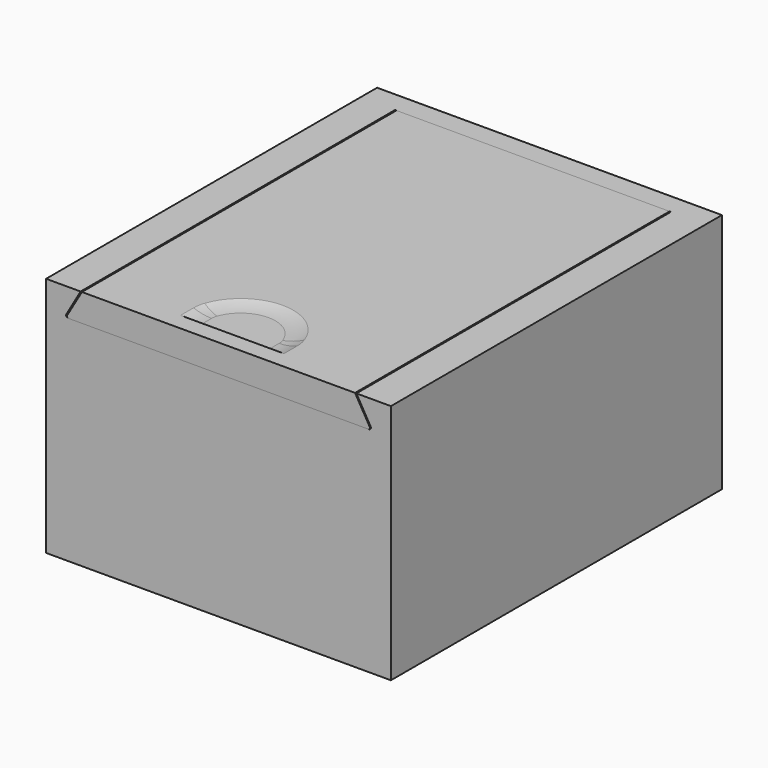
from build123d import *

# Parameters (mm, degrees)
F1_DEPTH      = 30
F1_DEPTH_BACK = 30
F2_W          = 40
F2_H          = 26
F3_DEPTH      = 3
F5_DEPTH      = 3
F6_DEPTH      = 30
F6_DEPTH_BACK = 27
F8_DEPTH      = 0.5
F9_T1_DEPTH   = 2.3744754405
F9_T4_ANGLE   = 141.4413290381
F9_T6_ANGLE   = 19.2793354809
F9_T8_ANGLE   = 19.2793354809


# Not quite as in the source:
# - a fillet or chamfer that OpenCascade refuses, or shapes differently, is made with other operations: its cross-section is extruded or revolved along the edge and cut away or added


with BuildPart() as f1:
    # F0 (on Front) → F1 (new body, two sides)
    with BuildSketch(Plane.XZ) as f1_sk:
        with BuildLine():
            Line((-25, -15), (0, -15))
            Line((0, -15), (0, -10))
            Line((0, -10), (-20, -10))
            Line((-20, -10), (-20, 15.9987840325))
            Line((-20, 15.9987840325), (-20, 16))
            Line((-20, 16), (-21.7897858345, 16))
            ThreePointArc((-21.7897858345, 16), (-22.0495934556, 16.15), (-22.0495934556, 16.45))
            Line((-22.0495934556, 16.45), (-20, 20))
            Line((-20, 20), (-25, 20))
            Line((-25, 20), (-25, -15))
        make_face()
        with BuildLine():
            Line((0, -10), (0, -15))
            Line((0, -15), (25, -15))
            Line((25, -15), (25, 20))
            Line((25, 20), (20, 20))
            Line((20, 20), (22.0495934556, 16.45))
            ThreePointArc((22.0495934556, 16.45), (22.0495934556, 16.15), (21.7897858345, 16))
            Line((21.7897858345, 16), (20, 16))
            Line((20, 16), (20, 15.9987840325))
            Line((20, 15.9987840325), (20, -10))
            Line((20, -10), (0, -10))
        make_face()
    extrude(amount=-F1_DEPTH)
    extrude(f1_sk.sketch, amount=F1_DEPTH_BACK)

    # F2 (on face) → F3 (join)
    with BuildSketch(Plane.XZ.offset(30)):
        with Locations((0, 3)):
            Rectangle(F2_W, F2_H)
        Polygon((-21.7897858345, 16), (-25, 16), (-25, -15), (25, -15), (25, 16), (21.7897858345, 16), (20, 16), (20, -10), (-20, -10), (-20, 16), align=None)
    extrude(amount=-F3_DEPTH)

    # F4 (on face) → F5 (join)
    with BuildSketch(Plane(origin=(0, 30, 0), x_dir=(-1, 0, 0), z_dir=(0, 1, 0))):
        with BuildLine():
            Line((20, 20), (-20, 20))
            Line((-20, 20), (-22.0495934556, 16.45))
            ThreePointArc((-22.0495934556, 16.45), (-22.0495934556, 16.15), (-21.7897858345, 16))
            Line((-21.7897858345, 16), (-20, 16))
            Line((-20, 16), (-20, -10))
            Line((-20, -10), (20, -10))
            Line((20, -10), (20, 16))
            Line((20, 16), (21.7897858345, 16))
            ThreePointArc((21.7897858345, 16), (22.0495934556, 16.15), (22.0495934556, 16.45))
            Line((22.0495934556, 16.45), (20, 20))
        make_face()
    extrude(amount=-F5_DEPTH)


with BuildPart() as f6:
    # F0 (on Front) → F6 (new body, two sides)
    with BuildSketch(Plane.XZ) as f6_sk:
        with BuildLine():
            Line((-21.7897858345, 16), (-20, 16))
            Line((-20, 16), (0, 16))
            Line((0, 16), (20, 16))
            Line((20, 16), (21.7897858345, 16))
            ThreePointArc((21.7897858345, 16), (21.9370082159, 16.1571086836), (21.9153242604, 16.3713220681))
            Line((21.9153242604, 16.3713220681), (19.8, 20))
            Line((19.8, 20), (0, 20))
            Line((0, 20), (-19.8, 20))
            Line((-19.8, 20), (-21.9153242604, 16.3713220681))
            ThreePointArc((-21.9153242604, 16.3713220681), (-21.9370082159, 16.1571086836), (-21.7897858345, 16))
        make_face()
    extrude(amount=F6_DEPTH)
    extrude(f6_sk.sketch, amount=-F6_DEPTH_BACK)

    # F7 (on face) → F8 (cut)
    with BuildSketch(Plane.XY.offset(20)):
        with BuildLine():
            Line((-7.5, -27.5), (7.5, -27.5))
            Line((7.5, -27.5), (7.5, -25.1255245595))
            ThreePointArc((7.5, -25.1255245595), (7.4294017066, -24.2882678396), (7.219600474, -23.474654678))
            ThreePointArc((7.219600474, -23.474654678), (0, -18.3514707296), (-7.219600474, -23.474654678))
            ThreePointArc((-7.219600474, -23.474654678), (-7.4294017066, -24.2882678396), (-7.5, -25.1255245595))
            Line((-7.5, -25.1255245595), (-7.5, -27.5))
        make_face()
    extrude(amount=-F8_DEPTH, mode=Mode.SUBTRACT)

    # F9: fillet of radius 7 on 1 edges, made by hand

    # F9_s2 → F9_t1 (join)
    with BuildSketch(Plane.XZ.offset(25.1255245595)):
        with BuildLine():
            ThreePointArc((-7.5, 20), (-6.2247994442, 19.6261364576), (-4.9019237886, 19.5))
            Line((-4.9019237886, 19.5), (-7.5, 19.5))
            Line((-7.5, 19.5), (-7.5, 20))
        make_face()
        with BuildLine():
            ThreePointArc((7.5, 20), (6.2247994442, 19.6261364576), (4.9019237886, 19.5))
            Line((4.9019237886, 19.5), (7.5, 19.5))
            Line((7.5, 19.5), (7.5, 20))
        make_face()
    extrude(amount=F9_T1_DEPTH)

    # F9_s3 → F9_t4 (revolve)
    with BuildSketch(Plane(origin=(8.1031041262, -23.1656137798, 0), x_dir=(0, 0, 1), z_dir=(0.3301739763, -0.9439200948, 0))):
        with BuildLine():
            ThreePointArc((20, 0.9359941133), (19.6261364576, 2.2111946691), (19.5, 3.5340703247))
            Line((19.5, 3.5340703247), (19.5, 0.9359941133))
            Line((19.5, 0.9359941133), (20, 0.9359941133))
        make_face()
    revolve(axis=Axis((0, -26, 19.5), (0, 0, 1)), revolution_arc=F9_T4_ANGLE)

    # F9_s5 → F9_t6 (revolve)
    with BuildSketch(Plane.XZ.offset(25.1255245595)):
        with BuildLine():
            ThreePointArc((7.5, 20), (6.2247994442, 19.6261364576), (4.9019237886, 19.5))
            Line((4.9019237886, 19.5), (7.5, 19.5))
            Line((7.5, 19.5), (7.5, 20))
        make_face()
    revolve(axis=Axis((2.5, -25.1255245595, 19.5), (0, 0, 1)), revolution_arc=F9_T6_ANGLE)

    # F9_s7 → F9_t8 (revolve)
    with BuildSketch(Plane(origin=(-8.1031041262, -23.1656137798, 0), x_dir=(0, 0, 1), z_dir=(0.3301739763, 0.9439200948, 0))):
        with BuildLine():
            ThreePointArc((20, 0.9359941133), (19.6261364576, 2.2111946691), (19.5, 3.5340703247))
            Line((19.5, 3.5340703247), (19.5, 0.9359941133))
            Line((19.5, 0.9359941133), (20, 0.9359941133))
        make_face()
    revolve(axis=Axis((-2.5, -25.1255245595, 19.5), (0, 0, 1)), revolution_arc=F9_T8_ANGLE)


solid = Compound([f1.part, f6.part])
